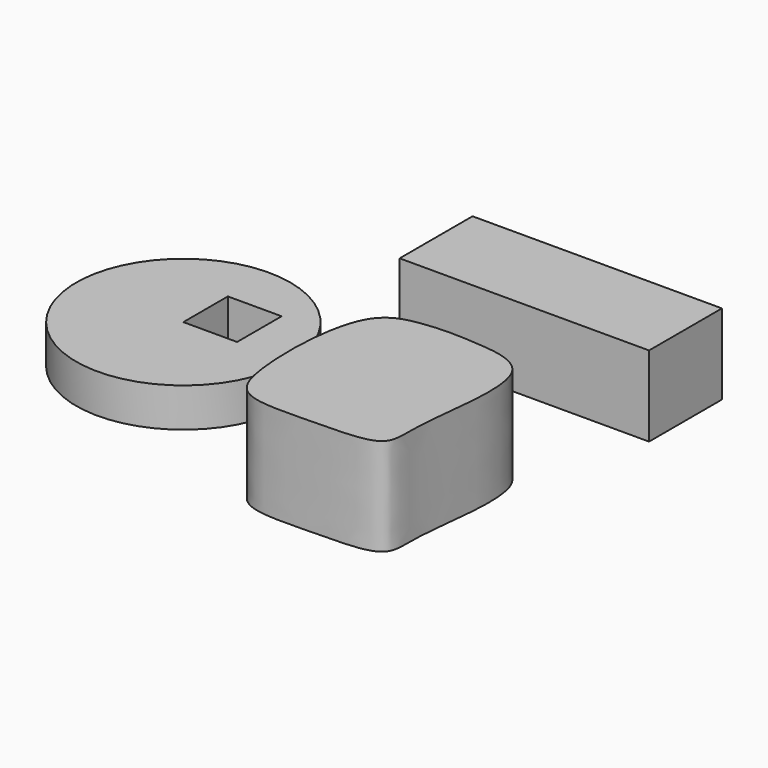
from build123d import *

# Parameters (mm, degrees)
F0_R     = 27.5
F0_W     = 13.7990014628
F0_H     = 14.2831781413
F1_DEPTH = 10
F2_W     = 63.9963464346
F2_H     = 23.3759097755
F3_DEPTH = 20.6
F9_DEPTH = 25


# Not quite as in the source:
# - the program builds the solid bodies; features that only make, move or delete a surface that nothing else refers to are left out


with BuildPart() as f1:
    # F0 (on Top) → F1 (new body)
    with BuildSketch(Plane.XY):
        with Locations((-25.5402568728, -16.2198804319)):
            Circle(F0_R)
        with Locations((-18.6407561414, -9.0782913612)):
            Rectangle(F0_W, F0_H, mode=Mode.SUBTRACT)
    extrude(amount=F1_DEPTH)


with BuildPart() as f3:
    # F2 (on Top) → F3 (new body)
    with BuildSketch(Plane.XY):
        with Locations((35.7344887452, 28.2618608326)):
            Rectangle(F2_W, F2_H)
    extrude(amount=F3_DEPTH)


with BuildPart() as f9:
    # F8 (on Top) → F9 (new body)
    with BuildSketch(Plane.XY):
        with BuildLine():
            add(Edge.make_bspline(
                [(29.4114947319, -9.4844894484), (26.3729347773, -9.9669040751), (16.9003945389, -12.2701929719), (16.0041992708, -44.345029821), (20.4782764199, -56.2412922253), (33.4595990445, -56.5220444535), (42.7791961025, -56.2278149781), (58.6401072937, -55.9435785579), (56.2352878094, -43.6996249686), (63.1171554107, -11.1002415527), (44.9569815233, -9.169865832), (36.6510831635, -8.7693531278), (31.9583329877, -9.0801426378), (29.4114947319, -9.4844894484)],
                knots=[0, 0, 0, 0, 0.0794581558, 0.2159553788, 0.3009189779, 0.3832422311, 0.4650488142, 0.5531355725, 0.6332820157, 0.7689335211, 0.8600368102, 0.9334003364, 1, 1, 1, 1], degree=3))
        make_face()
    extrude(amount=F9_DEPTH)


solid = Compound([f1.part, f3.part, f9.part])
